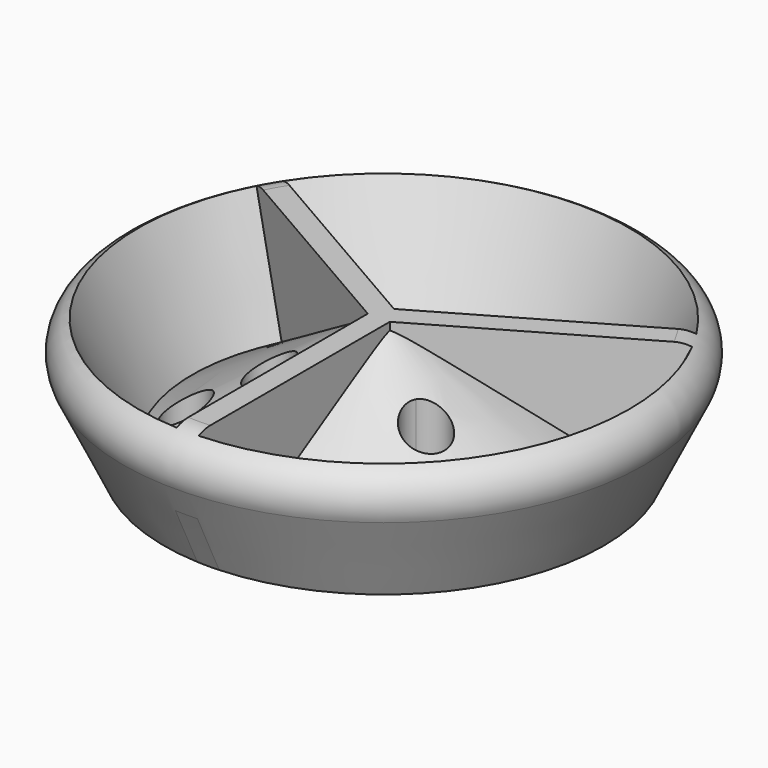
from build123d import *

# Parameters (mm, degrees)
F3_DEPTH = 6
F5_DEPTH = 6.0010001
F6_R     = 1
F7_DEPTH = 5


# Not quite as in the source:
# - a fillet or chamfer that OpenCascade refuses, or shapes differently, is made with other operations: its cross-section is extruded or revolved along the edge and cut away or added


with BuildPart() as f1:
    # F0 (on Front) → F1 (revolve)
    with BuildSketch(Plane.XZ):
        Polygon((0, 0), (10, 0), (8.7085954955, 0.7748427027), (0, 6), align=None)
        Polygon((8.7085954955, 0.7748427027), (10, 0), (12.905373238, 6), (11.2387675248, 6), align=None)
    revolve(axis=Axis((0, 0, 3), (0, 0, -1)))

    # F2 (on face) → F3 (join, through all)
    with BuildSketch(Plane.XY.offset(6)):
        with BuildLine():
            Line((0, -11.2387675248), (0, 0))
            Line((0, 0), (-9.7330581837, 5.6193837624))
            ThreePointArc((-9.7330581837, 5.6193837624), (-9.8556796151, 5.401432662), (-9.9734212913, 5.1808071981))
            Line((-9.9734212913, 5.1808071981), (-0.5, -0.2886751346))
            Line((-0.5, -0.2886751346), (-0.5, -11.2276397999))
            ThreePointArc((-0.5, -11.2276397999), (-0.2500619055, -11.2359852492), (0, -11.2387675248))
        make_face()
        with BuildLine():
            Line((9.7330581837, 5.6193837624), (0, 0))
            Line((0, 0), (0, -11.2387675248))
            ThreePointArc((0, -11.2387675248), (0.2500619055, -11.2359852492), (0.5, -11.2276397999))
            Line((0.5, -11.2276397999), (0.5, -0.2886751346))
            Line((0.5, -0.2886751346), (9.9734212913, 5.1808071981))
            ThreePointArc((9.9734212913, 5.1808071981), (9.8556796151, 5.401432662), (9.7330581837, 5.6193837624))
        make_face()
        with BuildLine():
            Line((-9.7330581837, 5.6193837624), (0, 0))
            Line((0, 0), (9.7330581837, 5.6193837624))
            ThreePointArc((9.7330581837, 5.6193837624), (9.6056177096, 5.8345525873), (9.4734212913, 6.0468326019))
            Line((9.4734212913, 6.0468326019), (0, 0.5773502692))
            Line((0, 0.5773502692), (-9.4734212913, 6.0468326019))
            ThreePointArc((-9.4734212913, 6.0468326019), (-9.6056177096, 5.8345525873), (-9.7330581837, 5.6193837624))
        make_face()
    extrude(amount=-F3_DEPTH)

    # F4 (on face) → F5 (cut, through all)
    with BuildSketch(Plane.XY.offset(6)):
        with BuildLine():
            ThreePointArc((7.1655671975, -3.5596918812), (6.4243862426, -2.5937660549), (5.2995417938, -3.0596918812))
            Line((5.2995417938, -3.0596918812), (7.0315926013, -4.0596918812))
            ThreePointArc((7.0315926013, -4.0596918812), (7.1314930238, -3.8185109263), (7.1655671975, -3.5596918812))
        make_face()
        with BuildLine():
            Line((7.0315926013, -4.0596918812), (5.2995417938, -3.0596918812))
            ThreePointArc((5.2995417938, -3.0596918812), (5.6655671975, -4.425717285), (7.0315926013, -4.0596918812))
        make_face()
        with BuildLine():
            ThreePointArc((4.5674909862, -2.0596918812), (3.8263100313, -1.0937660549), (2.7014655824, -1.5596918812))
            Line((2.7014655824, -1.5596918812), (4.43351639, -2.5596918812))
            ThreePointArc((4.43351639, -2.5596918812), (4.5334168125, -2.3185109263), (4.5674909862, -2.0596918812))
        make_face()
        with BuildLine():
            Line((4.43351639, -2.5596918812), (2.7014655824, -1.5596918812))
            ThreePointArc((2.7014655824, -1.5596918812), (3.0674909862, -2.925717285), (4.43351639, -2.5596918812))
        make_face()
        with BuildLine():
            ThreePointArc((-5.1655671975, -3.5596918812), (-5.1996413713, -3.3008728361), (-5.2995417938, -3.0596918812))
            Line((-5.2995417938, -3.0596918812), (-7.0315926013, -4.0596918812))
            ThreePointArc((-7.0315926013, -4.0596918812), (-5.9067481524, -4.5256177075), (-5.1655671975, -3.5596918812))
        make_face()
        with BuildLine():
            Line((-7.0315926013, -4.0596918812), (-5.2995417938, -3.0596918812))
            ThreePointArc((-5.2995417938, -3.0596918812), (-6.6655671975, -2.6936664774), (-7.0315926013, -4.0596918812))
        make_face()
        with BuildLine():
            ThreePointArc((-2.5674909862, -2.0596918812), (-2.6015651599, -1.8008728361), (-2.7014655824, -1.5596918812))
            Line((-2.7014655824, -1.5596918812), (-4.43351639, -2.5596918812))
            ThreePointArc((-4.43351639, -2.5596918812), (-3.3086719411, -3.0256177075), (-2.5674909862, -2.0596918812))
        make_face()
        with BuildLine():
            Line((-4.43351639, -2.5596918812), (-2.7014655824, -1.5596918812))
            ThreePointArc((-2.7014655824, -1.5596918812), (-4.0674909862, -1.1936664774), (-4.43351639, -2.5596918812))
        make_face()
        with BuildLine():
            ThreePointArc((0, 8.1193837624), (-1, 7.1193837624), (0, 6.1193837624))
            Line((0, 6.1193837624), (0, 8.1193837624))
        make_face()
        with BuildLine():
            Line((0, 8.1193837624), (0, 6.1193837624))
            ThreePointArc((0, 6.1193837624), (0.7071067812, 6.4122769812), (1, 7.1193837624))
            ThreePointArc((1, 7.1193837624), (0.7071067812, 7.8264905436), (0, 8.1193837624))
        make_face()
        with BuildLine():
            ThreePointArc((0, 5.1193837624), (-1, 4.1193837624), (0, 3.1193837624))
            Line((0, 3.1193837624), (0, 5.1193837624))
        make_face()
        with BuildLine():
            Line((0, 5.1193837624), (0, 3.1193837624))
            ThreePointArc((0, 3.1193837624), (0.7071067812, 3.4122769812), (1, 4.1193837624))
            ThreePointArc((1, 4.1193837624), (0.7071067812, 4.8264905436), (0, 5.1193837624))
        make_face()
    extrude(amount=-F5_DEPTH, mode=Mode.SUBTRACT)

    # F6 (on face) → F7 (cut)
    with BuildSketch(Plane(origin=(0, 0, 0), x_dir=(1, 0, 0), z_dir=(0, 0, -1))):
        Circle(F6_R)
    extrude(amount=-F7_DEPTH, mode=Mode.SUBTRACT)

    # F8: fillet of radius 1.5 on 1 edges, made by hand

    # F8_s1 → F8_t2 (revolve, cut)
    with BuildSketch(Plane.XZ):
        with BuildLine():
            ThreePointArc((11.8624735894, 3.8462671131), (11.7833686143, 5.2966808237), (10.5124242153, 6))
            Line((10.5124242153, 6), (12.905373238, 6))
            Line((12.905373238, 6), (11.8624735894, 3.8462671131))
        make_face()
    revolve(axis=Axis((0, 0, 6), (0, 0, -1)), mode=Mode.SUBTRACT)

    # F0 (on Front) → F9 (revolve, cut)
    with BuildSketch(Plane.XZ):
        Polygon((12.905373238, 6), (10, 0), (13.7833622578, 0), (16.6887354958, 6), align=None)
    revolve(axis=Axis((0, 0, 3), (0, 0, -1)), mode=Mode.SUBTRACT)


solid = f1.part
